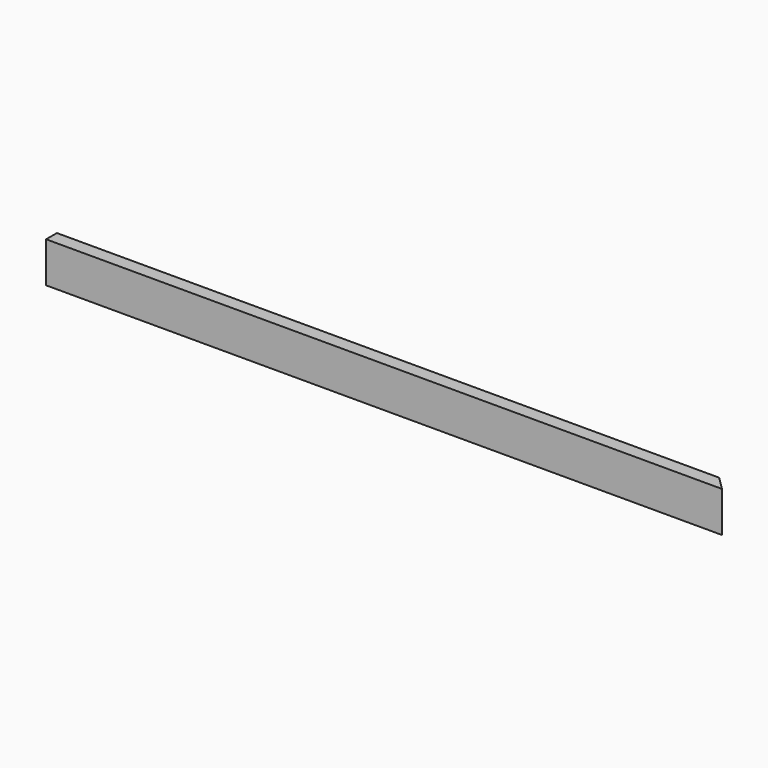
from build123d import *

# Parameters (mm, degrees)
F0_W        = 2540
F0_H        = 152.4
F1_DEPTH    = 50.8
F2_R        = 12.7
F3_DEPTH    = 2540
F4_T1_DEPTH = 413.6829915773


# Not quite as in the source:
# - a fillet or chamfer that OpenCascade refuses, or shapes differently, is made with other operations: its cross-section is extruded or revolved along the edge and cut away or added


with BuildPart() as f1:
    # F0 (on Front) → F1 (new body)
    with BuildSketch(Plane.XZ):
        with Locations((996.8233792729, 9.1693531722)):
            Rectangle(F0_W, F0_H)
    extrude(amount=F1_DEPTH)

    # F2 (on face) → F3 (cut)
    with BuildSketch(Plane(origin=(-273.1766207271, 0, 0), x_dir=(0, -1, 0), z_dir=(-1, 0, 0))):
        with Locations((25.4, 34.5693531722)):
            Circle(F2_R)
        with Locations((25.4, -16.2306468278)):
            Circle(F2_R)
    extrude(amount=-F3_DEPTH, mode=Mode.SUBTRACT)

    # F4: chamfer of 50.8 on 1 edges, made by hand

    # F4_s2 → F4_t1 (cut)
    with BuildSketch(Plane.XY.offset(-197.6721426165)):
        Polygon((2266.8233792729, -50.8), (2216.0233792729, 0), (2266.8233792729, 0), align=None)
    extrude(amount=F4_T1_DEPTH, mode=Mode.SUBTRACT)


solid = f1.part
